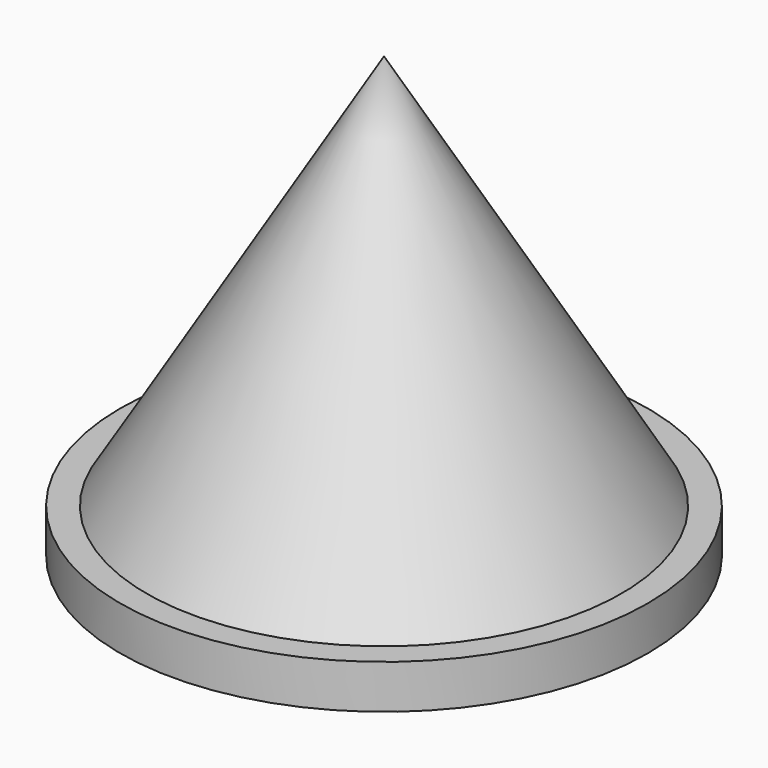
from build123d import *

# Parameters (mm, degrees)
F2_T = 2.54


# Not quite as in the source:
# - a shell that OpenCascade refuses in one call is made with other operations: the cavity is built on its own and cut out


with BuildPart() as f1:
    # F0 (on Front) → F1 (revolve)
    with BuildSketch(Plane.XZ):
        Polygon((-15.24, 0), (0, 0), (0, 2.54), (-13.716, 2.54), align=None)
        Polygon((-13.716, 2.54), (0, 2.54), (0, 25.4), align=None)
        Polygon((-15.24, 2.54), (-15.24, 0), (-13.716, 2.54), align=None)
    revolve(axis=Axis((0, 0, 12.7), (0, 0, 1)))

    # F2: shell of thickness 2.54, made by hand


with BuildPart() as f2_core1:
    # F2_t2: copy of F1
    add(f1.part)

    # the walls: a layer under each face that stays
    f2_faces = [f2_core1.faces().sort_by_distance(p)[0] for p in [
        (6.858, 0, 13.97),
        (-10.16, 10.16, 2.54),
        (15.24, 0, 1.27),
    ]]
    thicken(f2_faces, amount=-F2_T, mode=Mode.SUBTRACT)

    # F2_s3 → F2_t4 (revolve, cut)
    with BuildSketch(Plane.XZ):
        Polygon((-13.7377803203, 2.5784681922), (-11.5379679687, 1.2331807812), (-12.2778764374, 0), (-13.716, 0), align=None)
    revolve(axis=Axis((0, 0, 2.54), (0, 0, 1)), mode=Mode.SUBTRACT)


with BuildPart() as f1_1:
    add(f1.part)

    # what is left inside the walls is the cavity
    f2_cavity = [f2_core1.part.solids().sort_by_distance(p)[0] for p in [
        (3.824209, 0, 14.040077),
    ]]
    add(f2_cavity, mode=Mode.SUBTRACT)


solid = f1_1.part
